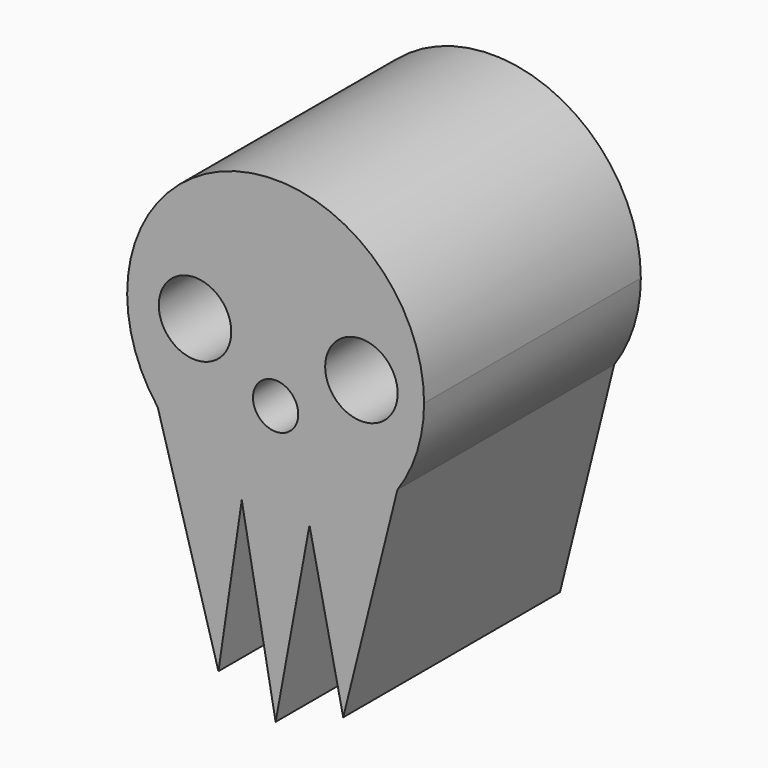
from build123d import *

# Parameters (mm, degrees)
F1_DEPTH     = 29.9
F3_D         = 8
F5_D         = 8
F7_D         = 5
F8_TEXT_SIZE = 8.3674883677
F9_DEPTH     = 1.1


# Not quite as in the source:
# - Text() gives the source's letters only with a copy of the font that has no kerning and outlines rounded to 1/6400 em; it was checked with that copy


with BuildPart() as f1:
    # F0 (on Front) → F1 (new body)
    with BuildSketch(Plane.XZ):
        with BuildLine():
            ThreePointArc((13.437245312, -9.372918063), (15.6294116368, -4.9124990054), (16.383258363, 0))
            ThreePointArc((16.383258363, 0), (-5.2630217704, 15.5148882186), (-13.0018311107, -9.9681263214))
            Line((-13.0018311107, -9.9681263214), (13.437245312, -9.372918063))
        make_face()
        with BuildLine():
            Line((13.437245312, -9.372918063), (-13.0018311107, -9.9681263214))
            ThreePointArc((-13.0018311107, -9.9681263214), (-8.8876771219, -13.7630065744), (-3.7362054716, -15.9515492434))
            ThreePointArc((-3.7362054716, -15.9515492434), (0, -16.383258363), (3.7362054716, -15.9515492434))
            ThreePointArc((3.7362054716, -15.9515492434), (9.195186241, -13.5594876225), (13.437245312, -9.372918063))
        make_face()
        with BuildLine():
            Line((7.4590169825, -33.4221310914), (13.437245312, -9.372918063))
            ThreePointArc((13.437245312, -9.372918063), (9.195186241, -13.5594876225), (3.7362054716, -15.9515492434))
            Line((3.7362054716, -15.9515492434), (7.4590169825, -33.4221310914))
        make_face()
        with BuildLine():
            ThreePointArc((3.7362054716, -15.9515492434), (0, -16.383258363), (-3.7362054716, -15.9515492434))
            Line((-3.7362054716, -15.9515492434), (0, -36.2909846008))
            Line((0, -36.2909846008), (3.7362054716, -15.9515492434))
        make_face()
        with BuildLine():
            ThreePointArc((-3.7362054716, -15.9515492434), (-8.8876771219, -13.7630065744), (-13.0018311107, -9.9681263214))
            Line((-13.0018311107, -9.9681263214), (-6.3114752993, -33.4221310914))
            Line((-6.3114752993, -33.4221310914), (-3.7362054716, -15.9515492434))
        make_face()
    extrude(amount=F1_DEPTH)

    # F3 (through all)
    with Locations(Plane(origin=(0, 0, 0), x_dir=(1, 0, 0), z_dir=(0, 1, 0))):
        with Locations((-8.8934432715, 0)):
            Hole(F3_D / 2)

    # F5 (through all)
    with Locations(Plane.XZ.offset(29.9)):
        with Locations((9.4672134146, 0)):
            Hole(F5_D / 2)

    # F7 (through all)
    with Locations(Plane.XZ.offset(29.9)):
        with Locations((0, -5.5942628533)):
            Hole(F7_D / 2)

    # F8 (on face) → F9 (join)
    with BuildSketch(Plane(origin=(0, 0, 0), x_dir=(-1, 0, 0), z_dir=(0, 1, 0))):
        with Locations((-8.8934416417, 5.8811465278)):
            Text('Kaia', F8_TEXT_SIZE, font='Open Sans', text_align=(TextAlign.LEFT, TextAlign.BOTTOM))
    extrude(amount=F9_DEPTH)


solid = f1.part
